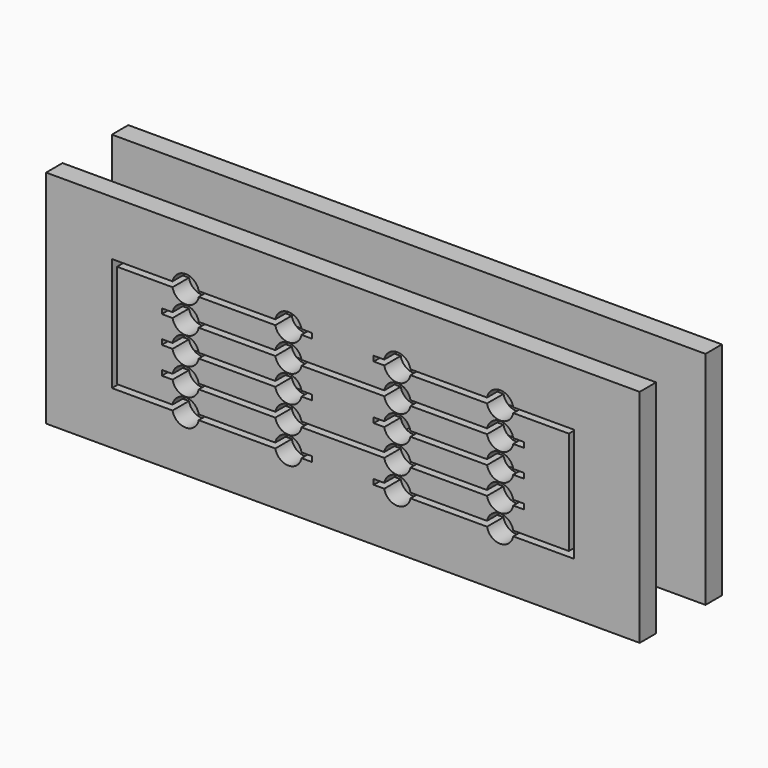
from build123d import *

# Parameters (mm, degrees)
F1_DEPTH = 10
F2_DEPTH = 25
F4_W     = 30
F4_H     = 30
F5_DEPTH = 0.1


with BuildPart() as f1:
    # F0 (on Front) → F1 (new body)
    with BuildSketch(Plane.XZ):
        with BuildLine():
            Line((-112.3982608318, 0), (112.3982608318, 0))
            Line((112.3982608318, 0), (112.3982608318, 25.6207627171))
            Line((112.3982608318, 25.6207627171), (82.8786754111, 25.6207627171))
            ThreePointArc((82.8786754111, 25.6207627171), (76.5, 20.3707627171), (70.1213245889, 25.6207627171))
            Line((70.1213245889, 25.6207627171), (32.8786754111, 25.6207627171))
            ThreePointArc((32.8786754111, 25.6207627171), (26.5, 20.3707627171), (20.1213245889, 25.6207627171))
            Line((20.1213245889, 25.6207627171), (15, 25.6207627171))
            Line((15, 25.6207627171), (-15, 25.6207627171))
            Line((-15, 25.6207627171), (-20.1213245889, 25.6207627171))
            ThreePointArc((-20.1213245889, 25.6207627171), (-26.5, 20.3707627171), (-32.8786754111, 25.6207627171))
            Line((-32.8786754111, 25.6207627171), (-70.1213245889, 25.6207627171))
            ThreePointArc((-70.1213245889, 25.6207627171), (-76.5, 20.3707627171), (-82.8786754111, 25.6207627171))
            Line((-82.8786754111, 25.6207627171), (-112.3982608318, 25.6207627171))
            Line((-112.3982608318, 25.6207627171), (-112.3982608318, 0))
        make_face()
        Polygon((112.3982608318, 25.6207627171), (112.3982608318, 0), (144.3929672241, 0), (144.3929672241, 107.523843646), (112.3982608318, 107.523843646), (112.3982608318, 80.9207627171), align=None)
        Polygon((-144.3929672241, 0), (-112.3982608318, 0), (-112.3982608318, 25.6207627171), (-112.3982608318, 80.9207627171), (-112.3982608318, 107.523843646), (-144.3929672241, 107.523843646), align=None)
        with BuildLine():
            Line((82.8786754111, 80.9207627171), (112.3982608318, 80.9207627171))
            Line((112.3982608318, 80.9207627171), (112.3982608318, 107.523843646))
            Line((112.3982608318, 107.523843646), (-112.3982608318, 107.523843646))
            Line((-112.3982608318, 107.523843646), (-112.3982608318, 80.9207627171))
            Line((-112.3982608318, 80.9207627171), (-82.8786754111, 80.9207627171))
            ThreePointArc((-82.8786754111, 80.9207627171), (-76.5, 86.1707627171), (-70.1213245889, 80.9207627171))
            Line((-70.1213245889, 80.9207627171), (-32.8786754111, 80.9207627171))
            ThreePointArc((-32.8786754111, 80.9207627171), (-26.5, 86.1707627171), (-20.1213245889, 80.9207627171))
            Line((-20.1213245889, 80.9207627171), (-15, 80.9207627171))
            Line((-15, 80.9207627171), (15, 80.9207627171))
            Line((15, 80.9207627171), (20.1213245889, 80.9207627171))
            ThreePointArc((20.1213245889, 80.9207627171), (26.5, 86.1707627171), (32.8786754111, 80.9207627171))
            Line((32.8786754111, 80.9207627171), (70.1213245889, 80.9207627171))
            ThreePointArc((70.1213245889, 80.9207627171), (76.5, 86.1707627171), (82.8786754111, 80.9207627171))
        make_face()
        with BuildLine():
            Line((-88.1, 28.1207627171), (-82.8786754111, 28.1207627171))
            ThreePointArc((-82.8786754111, 28.1207627171), (-76.5, 33.3707627171), (-70.1213245889, 28.1207627171))
            Line((-70.1213245889, 28.1207627171), (-32.8786754111, 28.1207627171))
            ThreePointArc((-32.8786754111, 28.1207627171), (-26.5, 33.3707627171), (-20.1213245889, 28.1207627171))
            Line((-20.1213245889, 28.1207627171), (-15, 28.1207627171))
            Line((-15, 28.1207627171), (-15, 38.8207627171))
            Line((-15, 38.8207627171), (-20.1213245889, 38.8207627171))
            ThreePointArc((-20.1213245889, 38.8207627171), (-26.5, 33.5707627171), (-32.8786754111, 38.8207627171))
            Line((-32.8786754111, 38.8207627171), (-70.1213245889, 38.8207627171))
            ThreePointArc((-70.1213245889, 38.8207627171), (-76.5, 33.5707627171), (-82.8786754111, 38.8207627171))
            Line((-82.8786754111, 38.8207627171), (-88.1, 38.8207627171))
            Line((-88.1, 38.8207627171), (-88.1, 28.1207627171))
        make_face()
        with BuildLine():
            Line((32.8786754111, 28.1207627171), (70.1213245889, 28.1207627171))
            ThreePointArc((70.1213245889, 28.1207627171), (76.5, 33.3707627171), (82.8786754111, 28.1207627171))
            Line((82.8786754111, 28.1207627171), (88.1, 28.1207627171))
            Line((88.1, 28.1207627171), (88.1, 38.8207627171))
            Line((88.1, 38.8207627171), (82.8786754111, 38.8207627171))
            ThreePointArc((82.8786754111, 38.8207627171), (76.5, 33.5707627171), (70.1213245889, 38.8207627171))
            Line((70.1213245889, 38.8207627171), (32.8786754111, 38.8207627171))
            ThreePointArc((32.8786754111, 38.8207627171), (26.5, 33.5707627171), (20.1213245889, 38.8207627171))
            Line((20.1213245889, 38.8207627171), (15, 38.8207627171))
            Line((15, 38.8207627171), (15, 28.1207627171))
            Line((15, 28.1207627171), (20.1213245889, 28.1207627171))
            ThreePointArc((20.1213245889, 28.1207627171), (26.5, 33.3707627171), (32.8786754111, 28.1207627171))
        make_face()
        Polygon((-109.8982608318, 28.1207627171), (-88.1, 28.1207627171), (-88.1, 38.8207627171), (-88.1, 41.3207627171), (-88.1, 52.0207627171), (-88.1, 54.5207627171), (-88.1, 65.2207627171), (-88.1, 67.7207627171), (-88.1, 78.4207627171), (-109.8982608318, 78.4207627171), align=None)
        with BuildLine():
            ThreePointArc((-70.1213245889, 78.4207627171), (-76.5, 73.1707627171), (-82.8786754111, 78.4207627171))
            Line((-82.8786754111, 78.4207627171), (-88.1, 78.4207627171))
            Line((-88.1, 78.4207627171), (-88.1, 67.7207627171))
            Line((-88.1, 67.7207627171), (-82.8786754111, 67.7207627171))
            ThreePointArc((-82.8786754111, 67.7207627171), (-76.5, 72.9707627171), (-70.1213245889, 67.7207627171))
            Line((-70.1213245889, 67.7207627171), (-32.8786754111, 67.7207627171))
            ThreePointArc((-32.8786754111, 67.7207627171), (-26.5, 72.9707627171), (-20.1213245889, 67.7207627171))
            Line((-20.1213245889, 67.7207627171), (-15, 67.7207627171))
            Line((-15, 67.7207627171), (-15, 78.4207627171))
            Line((-15, 78.4207627171), (-20.1213245889, 78.4207627171))
            ThreePointArc((-20.1213245889, 78.4207627171), (-26.5, 73.1707627171), (-32.8786754111, 78.4207627171))
            Line((-32.8786754111, 78.4207627171), (-70.1213245889, 78.4207627171))
        make_face()
        Polygon((88.1, 38.8207627171), (88.1, 28.1207627171), (109.8982608318, 28.1207627171), (109.8982608318, 78.4207627171), (88.1, 78.4207627171), (88.1, 67.7207627171), (88.1, 65.2207627171), (88.1, 54.5207627171), (88.1, 52.0207627171), (88.1, 41.3207627171), align=None)
        with BuildLine():
            ThreePointArc((82.8786754111, 78.4207627171), (76.5, 73.1707627171), (70.1213245889, 78.4207627171))
            Line((70.1213245889, 78.4207627171), (32.8786754111, 78.4207627171))
            ThreePointArc((32.8786754111, 78.4207627171), (26.5, 73.1707627171), (20.1213245889, 78.4207627171))
            Line((20.1213245889, 78.4207627171), (15, 78.4207627171))
            Line((15, 78.4207627171), (15, 67.7207627171))
            Line((15, 67.7207627171), (20.1213245889, 67.7207627171))
            ThreePointArc((20.1213245889, 67.7207627171), (26.5, 72.9707627171), (32.8786754111, 67.7207627171))
            Line((32.8786754111, 67.7207627171), (70.1213245889, 67.7207627171))
            ThreePointArc((70.1213245889, 67.7207627171), (76.5, 72.9707627171), (82.8786754111, 67.7207627171))
            Line((82.8786754111, 67.7207627171), (88.1, 67.7207627171))
            Line((88.1, 67.7207627171), (88.1, 78.4207627171))
            Line((88.1, 78.4207627171), (82.8786754111, 78.4207627171))
        make_face()
        Polygon((-15, 25.6207627171), (15, 25.6207627171), (15, 28.1207627171), (15, 38.8207627171), (-15, 38.8207627171), (-15, 28.1207627171), align=None)
        with BuildLine():
            Line((-88.1, 52.0207627171), (-88.1, 41.3207627171))
            Line((-88.1, 41.3207627171), (-82.8786754111, 41.3207627171))
            ThreePointArc((-82.8786754111, 41.3207627171), (-76.5, 46.5707627171), (-70.1213245889, 41.3207627171))
            Line((-70.1213245889, 41.3207627171), (-32.8786754111, 41.3207627171))
            ThreePointArc((-32.8786754111, 41.3207627171), (-26.5, 46.5707627171), (-20.1213245889, 41.3207627171))
            Line((-20.1213245889, 41.3207627171), (-15, 41.3207627171))
            Line((-15, 41.3207627171), (-15, 52.0207627171))
            Line((-15, 52.0207627171), (-20.1213245889, 52.0207627171))
            ThreePointArc((-20.1213245889, 52.0207627171), (-26.5, 46.7707627171), (-32.8786754111, 52.0207627171))
            Line((-32.8786754111, 52.0207627171), (-70.1213245889, 52.0207627171))
            ThreePointArc((-70.1213245889, 52.0207627171), (-76.5, 46.7707627171), (-82.8786754111, 52.0207627171))
            Line((-82.8786754111, 52.0207627171), (-88.1, 52.0207627171))
        make_face()
        with BuildLine():
            Line((82.8786754111, 41.3207627171), (88.1, 41.3207627171))
            Line((88.1, 41.3207627171), (88.1, 52.0207627171))
            Line((88.1, 52.0207627171), (82.8786754111, 52.0207627171))
            ThreePointArc((82.8786754111, 52.0207627171), (76.5, 46.7707627171), (70.1213245889, 52.0207627171))
            Line((70.1213245889, 52.0207627171), (32.8786754111, 52.0207627171))
            ThreePointArc((32.8786754111, 52.0207627171), (26.5, 46.7707627171), (20.1213245889, 52.0207627171))
            Line((20.1213245889, 52.0207627171), (15, 52.0207627171))
            Line((15, 52.0207627171), (15, 41.3207627171))
            Line((15, 41.3207627171), (20.1213245889, 41.3207627171))
            ThreePointArc((20.1213245889, 41.3207627171), (26.5, 46.5707627171), (32.8786754111, 41.3207627171))
            Line((32.8786754111, 41.3207627171), (70.1213245889, 41.3207627171))
            ThreePointArc((70.1213245889, 41.3207627171), (76.5, 46.5707627171), (82.8786754111, 41.3207627171))
        make_face()
        Polygon((15, 78.4207627171), (15, 80.9207627171), (-15, 80.9207627171), (-15, 78.4207627171), (-15, 67.7207627171), (15, 67.7207627171), align=None)
        with BuildLine():
            Line((-82.8786754111, 65.2207627171), (-88.1, 65.2207627171))
            Line((-88.1, 65.2207627171), (-88.1, 54.5207627171))
            Line((-88.1, 54.5207627171), (-82.8786754111, 54.5207627171))
            ThreePointArc((-82.8786754111, 54.5207627171), (-76.5, 59.7707627171), (-70.1213245889, 54.5207627171))
            Line((-70.1213245889, 54.5207627171), (-32.8786754111, 54.5207627171))
            ThreePointArc((-32.8786754111, 54.5207627171), (-26.5, 59.7707627171), (-20.1213245889, 54.5207627171))
            Line((-20.1213245889, 54.5207627171), (-15, 54.5207627171))
            Line((-15, 54.5207627171), (-15, 65.2207627171))
            Line((-15, 65.2207627171), (-20.1213245889, 65.2207627171))
            ThreePointArc((-20.1213245889, 65.2207627171), (-26.5, 59.9707627171), (-32.8786754111, 65.2207627171))
            Line((-32.8786754111, 65.2207627171), (-70.1213245889, 65.2207627171))
            ThreePointArc((-70.1213245889, 65.2207627171), (-76.5, 59.9707627171), (-82.8786754111, 65.2207627171))
        make_face()
        with BuildLine():
            Line((88.1, 54.5207627171), (88.1, 65.2207627171))
            Line((88.1, 65.2207627171), (82.8786754111, 65.2207627171))
            ThreePointArc((82.8786754111, 65.2207627171), (76.5, 59.9707627171), (70.1213245889, 65.2207627171))
            Line((70.1213245889, 65.2207627171), (32.8786754111, 65.2207627171))
            ThreePointArc((32.8786754111, 65.2207627171), (26.5, 59.9707627171), (20.1213245889, 65.2207627171))
            Line((20.1213245889, 65.2207627171), (15, 65.2207627171))
            Line((15, 65.2207627171), (15, 54.5207627171))
            Line((15, 54.5207627171), (20.1213245889, 54.5207627171))
            ThreePointArc((20.1213245889, 54.5207627171), (26.5, 59.7707627171), (32.8786754111, 54.5207627171))
            Line((32.8786754111, 54.5207627171), (70.1213245889, 54.5207627171))
            ThreePointArc((70.1213245889, 54.5207627171), (76.5, 59.7707627171), (82.8786754111, 54.5207627171))
            Line((82.8786754111, 54.5207627171), (88.1, 54.5207627171))
        make_face()
    extrude(amount=F1_DEPTH)

    # F0 (on Front) → F2 (join)
    with BuildSketch(Plane.XZ):
        Polygon((-15, 41.3207627171), (15, 41.3207627171), (15, 52.0207627171), (15, 54.5207627171), (15, 65.2207627171), (-15, 65.2207627171), (-15, 54.5207627171), (-15, 52.0207627171), align=None)
    extrude(amount=F2_DEPTH)

    # F3: F1 across face


with BuildPart() as f1_1:
    add(f1.part)
    add(f1.part.mirror(Plane(origin=(0, -25, 53.2707627171), x_dir=(1, 0, 0), z_dir=(0, -1, 0))))

    # F4 (on face) → F5 (join)
    with BuildSketch(Plane(origin=(0, 0, 41.3207627171), x_dir=(1, 0, 0), z_dir=(0, 0, -1))):
        with Locations((0, 25)):
            Rectangle(F4_W, F4_H)
    extrude(amount=F5_DEPTH)


solid = f1_1.part
